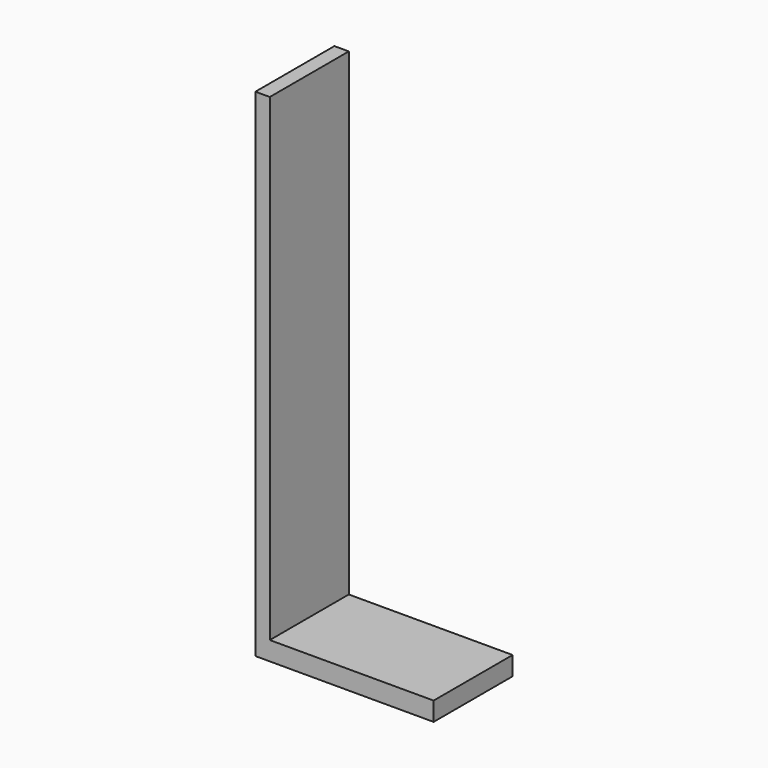
from build123d import *

# Parameters (mm, degrees)
F3_DEPTH = 12.7


# Not quite as in the source:
# - the program builds the solid bodies; features that only make, move or delete a surface that nothing else refers to are left out


with BuildPart() as f3:
    # F2 (on Front) → F3 (new body, symmetric)
    with BuildSketch(Plane.XZ):
        Polygon((59.2198967934, 63.1065145135), (55.5164813995, 63.1065145135), (55.5164813995, -59.8734021187), (55.5164813995, -64.7067055106), (101.3612598181, -64.7067055106), (101.3612598181, -59.8734021187), (59.2198967934, -59.8734021187), align=None)
    extrude(amount=F3_DEPTH, both=True)


solid = f3.part
